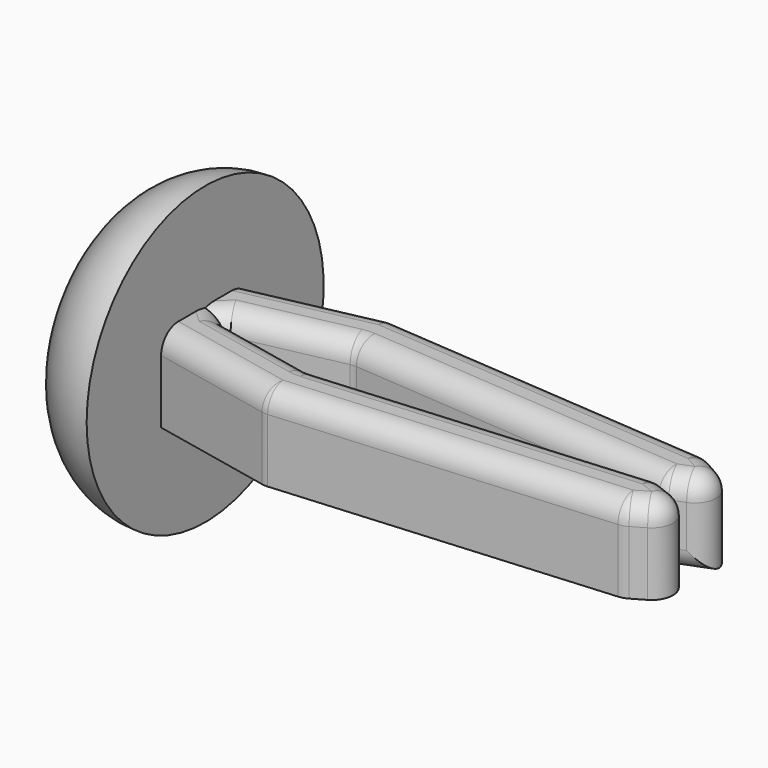
from build123d import *

# Parameters (mm, degrees)
F1_DEPTH = 2
F4_R     = 0.5
F4_2_R   = 0.5
F5_R     = 3.5
F6_DEPTH = 2
F7_R     = 1.99999


# Not quite as in the source:
# - a fillet or chamfer is up to 0.001 mm smaller than in the source, because OpenCascade refuses the exact size


with BuildPart() as f1:
    # F0 (on Top) → F1 (new body)
    with BuildSketch(Plane.XY):
        Polygon((2.93560655, 0.6182347319), (0, 0), (0, -1.7093243077), (0.5313075392, -1.2166232651), (3.0210481864, -0.6922872837), (10.8112192467, -1.2961123241), (12.209258666, -0.7525262849), (10.9116823906, 0), align=None)
    extrude(amount=F1_DEPTH)


with BuildPart() as f3_1:
    # F3: instance of F1
    add(f1.part.mirror(Plane.XZ.offset(1.3)))

    # F4#2
    f4_2_edges = [f3_1.edges().sort_by_distance(p)[0] for p in [
        (3.021048, -1.907713, 1),
        (10.811219, -1.303888, 1),
        (12.209259, -1.847474, 1),
        (10.911682, -2.6, 1),
        (6.923644, -2.909117, 2),
        (11.560471, -2.223737, 2),
        (6.916134, -1.6058, 2),
        (11.510239, -1.575681, 2),
        (1.467803, -2.909117, 2),
        (2.935607, -3.218235, 1),
        (1.776178, -1.645545, 2),
        (0.265654, -1.137026, 2),
    ]]
    fillet(f4_2_edges, radius=F4_2_R)


with BuildPart() as f1_1:
    add(f1.part)

    # F4
    f4_edges = [f1_1.edges().sort_by_distance(p)[0] for p in [
        (6.916134, -0.9942, 2),
        (6.923644, 0.309117, 2),
        (11.560471, -0.376263, 2),
        (10.811219, -1.296112, 1),
        (12.209259, -0.752526, 1),
        (11.510239, -1.024319, 0),
        (11.510239, -1.024319, 2),
        (1.467803, 0.309117, 2),
        (1.776178, -0.954455, 2),
        (3.021048, -0.692287, 1),
        (0.265654, -1.462974, 2),
        (10.911682, 0, 1),
        (2.935607, 0.618235, 1),
    ]]
    fillet(f4_edges, radius=F4_R)


with BuildPart() as f6:
    # F5 (on face) → F6 (new body)
    with BuildSketch(Plane(origin=(0, 0, 0), x_dir=(0, -1, 0), z_dir=(-1, 0, 0))):
        with Locations((1.3, 1)):
            Circle(F5_R)
        with BuildLine():
            Line((0, 0), (0, 1.5))
            add(Edge.make_bspline(
                [(0, 1.5), (0, 2), (0.5109676568, 2)],
                knots=[3.1415926536, 3.1415926536, 3.1415926536, 4.7123889804, 4.7123889804, 4.7123889804], degree=2, weights=[1, 0.7071067812, 1]))
            Line((0.5109676568, 2), (1.0274237333, 2))
            add(Edge.make_bspline(
                [(1.7093243077, 1.5), (1.7093243077, 2), (1.0274237333, 2)],
                knots=[3.1415926536, 3.1415926536, 3.1415926536, 4.7123889804, 4.7123889804, 4.7123889804], degree=2, weights=[1, 0.7071067812, 1]))
            Line((1.7093243077, 1.5), (1.7093243077, 0))
            Line((1.7093243077, 0), (0, 0))
        make_face(mode=Mode.SUBTRACT)
        with BuildLine():
            add(Edge.make_bspline(
                [(0, 1.5), (0, 2), (0.5109676568, 2)],
                knots=[3.1415926536, 3.1415926536, 3.1415926536, 4.7123889804, 4.7123889804, 4.7123889804], degree=2, weights=[1, 0.7071067812, 1]))
            Line((0, 1.5), (0, 0))
            Line((0, 0), (1.7093243077, 0))
            Line((1.7093243077, 0), (1.7093243077, 1.5))
            add(Edge.make_bspline(
                [(1.7093243077, 1.5), (1.7093243077, 2), (1.0274237333, 2)],
                knots=[3.1415926536, 3.1415926536, 3.1415926536, 4.7123889804, 4.7123889804, 4.7123889804], degree=2, weights=[1, 0.7071067812, 1]))
            Line((1.0274237333, 2), (0.5109676568, 2))
        make_face()
    extrude(amount=F6_DEPTH)

    # F7 (radius 2 in the source; OpenCascade refuses exactly that, so slightly less here)
    f7_edges = [f6.edges().sort_by_distance(p)[0] for p in [
        (-2, 2.2, 1),
    ]]
    fillet(f7_edges, radius=F7_R)


solid = Compound([f3_1.part, f1_1.part, f6.part])
